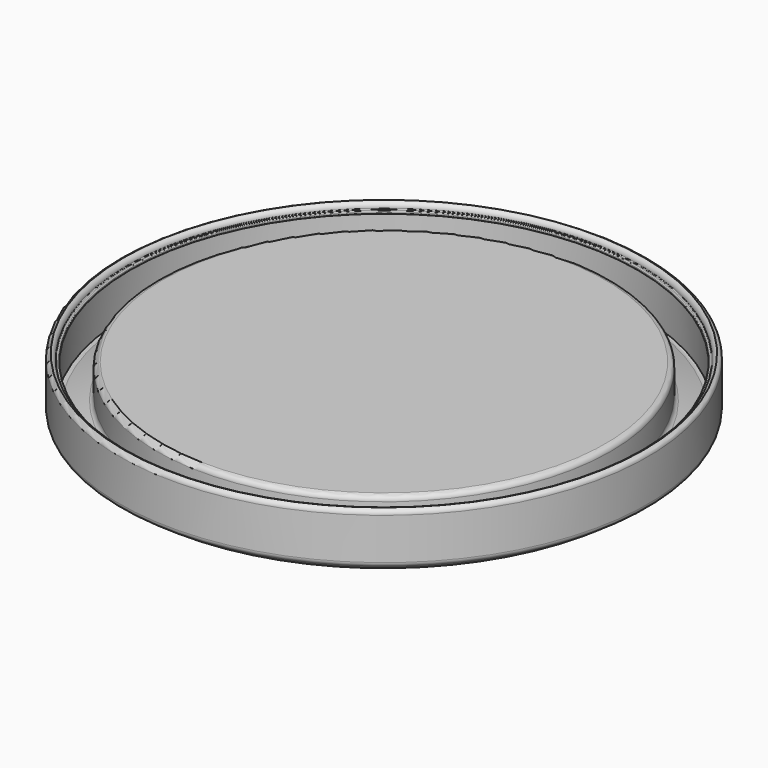
from build123d import *

# Parameters (mm, degrees)
F2_TEXT_SIZE = 19.8757763975
F3_DEPTH     = 2


# Not quite as in the source:
# - Text() gives the source's letters only with a copy of the font that has no kerning and outlines rounded to 1/6400 em; it was checked with that copy


with BuildPart() as f1:
    # F0 (on Front) → F1 (revolve)
    with BuildSketch(Plane.XZ):
        with BuildLine():
            ThreePointArc((-34.9908136561, 7.97342394), (-35.3583839629, 7.7219634897), (-35.5, 7.2997251842))
            Line((-35.5, 7.2997251842), (-35.5, 1.7109215066))
            ThreePointArc((-35.5, 1.7109215066), (-35.4188035947, 1.3836192925), (-35.1940437184, 1.1322180323))
            Line((-35.1940437184, 1.1322180323), (-33.7108145509, 0.1215713415))
            ThreePointArc((-33.7108145509, 0.1215713415), (-33.5228129437, 0.0310826586), (-33.3164960167, 0))
            Line((-33.3164960167, 0), (-30.5, 0))
            Line((-30.5, 0), (0, 0))
            Line((0, 0), (0, 2.1949816797))
            Line((0, 2.1949816797), (0, 7))
            Line((0, 7), (-29.7997251842, 7))
            ThreePointArc((-29.7997251842, 7), (-30.2948942552, 6.7948942552), (-30.5, 6.2997251842))
            Line((-30.5, 6.2997251842), (-30.5, 3.0779467612))
            ThreePointArc((-30.5, 3.0779467612), (-30.617813517, 2.6892005032), (-30.9316124175, 2.431258789))
            Line((-30.9316124175, 2.431258789), (-33.9299264837, 1.1856283114))
            ThreePointArc((-33.9299264837, 1.1856283114), (-34.2165166306, 1.1322709897), (-34.5, 1.2002275592))
            Line((-34.5, 1.2002275592), (-34.5, 6.6271514663))
            ThreePointArc((-34.5, 6.6271514663), (-34.4668316346, 6.7072269838), (-34.3867561171, 6.7403953492))
            Line((-34.3867561171, 6.7403953492), (-34.2132438829, 6.7403953492))
            ThreePointArc((-34.2132438829, 6.7403953492), (-34.1331683654, 6.7735637145), (-34.1, 6.853639232))
            Line((-34.1, 6.853639232), (-34.1, 7.0271253934))
            ThreePointArc((-34.1, 7.0271253934), (-34.1331683654, 7.1072009109), (-34.2132438829, 7.1403692762))
            Line((-34.2132438829, 7.1403692762), (-34.3946765933, 7.1403692762))
            ThreePointArc((-34.3946765933, 7.1403692762), (-34.4610500453, 7.1695863438), (-34.4843293277, 7.2382678345))
            ThreePointArc((-34.4843293277, 7.2382678345), (-34.6052364198, 7.6970178705), (-34.9908136561, 7.97342394))
        make_face()
    revolve(axis=Axis((0, 0, 1.0974908398), (0, 0, -1)))

    # F2 (on face) → F3 (cut)
    with BuildSketch(Plane(origin=(0, 0, 0), x_dir=(1, 0, 0), z_dir=(0, 0, -1))):
        with Locations((-25, -6.803585314)):
            Text('2o3A', F2_TEXT_SIZE, font='Open Sans', font_style=FontStyle.BOLD, text_align=(TextAlign.LEFT, TextAlign.BOTTOM))
    extrude(amount=-F3_DEPTH, mode=Mode.SUBTRACT)


solid = f1.part
